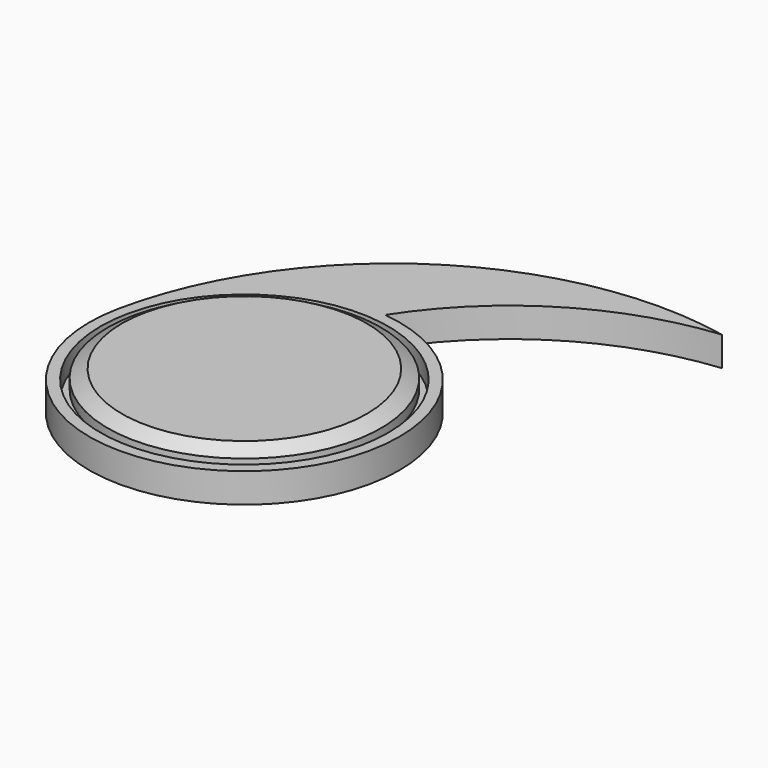
from build123d import *

# Parameters (mm, degrees)
F0_R     = 5
F0_R_2   = 1.5
F1_DEPTH = 2
F4_W     = 1.5
F4_H     = 2
F7_DEPTH = 4


# Not quite as in the source:
# - a feature of the source that left no trace in its solid (it failed there, or was rolled back) is left out


with BuildPart() as f1:
    # F0 (on Top) → F1 (new body)
    with BuildSketch(Plane.XY):
        Circle(F0_R)
        Circle(F0_R_2, mode=Mode.SUBTRACT)
    extrude(amount=F1_DEPTH)


with BuildPart() as f3:
    # F2 (on Front) → F3 (revolve)
    with BuildSketch(Plane.XZ):
        Polygon((-21, 0), (-5, 0), (-5, 2), (-7, 2), (-7, 1.5), (-19.5, 1.5), (-19.5, 4), (-21, 4), align=None)
    revolve(axis=Axis((0, 0, 2.9167793691), (0, 0, 1)))

    # F6 (on Top) → F7 (join, through all)
    with BuildSketch(Plane.XY):
        with BuildLine():
            ThreePointArc((2.3821237217, 20.8644550989), (15.5620656061, 33.7338722927), (33.0265901225, 39.5924685753))
            ThreePointArc((33.0265901225, 39.5924685753), (-1.0497554808, 32.9939806535), (-20.5580313112, 4.2857144807))
            ThreePointArc((-20.5580313112, 4.2857144807), (-12.3005920304, 17.0204417012), (2.3821237217, 20.8644550989))
        make_face()
    extrude(amount=F7_DEPTH)


with BuildPart() as f5:
    # F4 (on Front) → F5 (revolve)
    with BuildSketch(Plane.XZ):
        Polygon((0, 2), (0, 5.3), (-16.5947441117, 5.3), (-18.5, 4.2), (-18.5, 2.8428932188), (-17.2009618943, 2.0928932188), (-7.5, 2.0928932188), (-6.7928932188, 2.8), (-3.5, 2.8), (-3.5, 2), (-1.5, 2), align=None)
        with Locations((-0.75, 1)):
            Rectangle(F4_W, F4_H)
    revolve(axis=Axis((0, 0, 2.65), (0, 0, 1)))


solid = Compound([f1.part, f3.part, f5.part])
